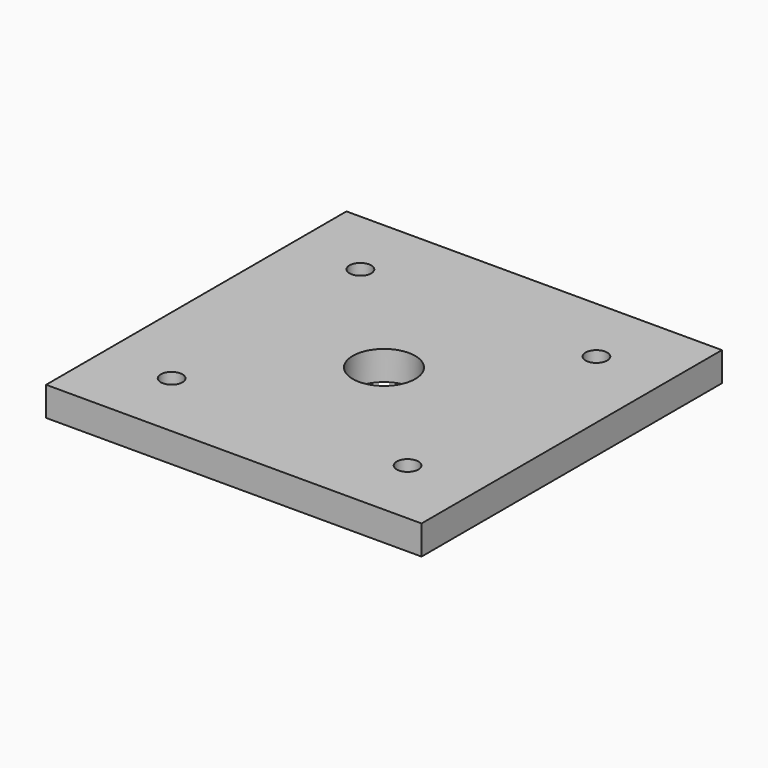
from build123d import *

# Parameters (mm, degrees)
F0_W     = 90
F0_H     = 90
F0_R     = 2.6
F0_R_2   = 2.5
F0_R_3   = 7.5
F1_DEPTH = 7
F2_DEPTH = 10


# Not quite as in the source:
# - a feature names something its author has since deleted; it is built from what else it names


with BuildPart() as f1:
    # F0 (on Top) → F1 (new body)
    with BuildSketch(Plane.XY):
        Rectangle(F0_W, F0_H)
        with Locations((-28.2842712475, -28.2842712475)):
            Circle(F0_R, mode=Mode.SUBTRACT)
        with Locations((-29.9999999986, -0.0002877)):
            Circle(F0_R_2, mode=Mode.SUBTRACT)
        with Locations((28.2842712475, -28.2842712475)):
            Circle(F0_R, mode=Mode.SUBTRACT)
        with Locations((-28.2842712475, 28.2842712475)):
            Circle(F0_R, mode=Mode.SUBTRACT)
        Circle(F0_R_3, mode=Mode.SUBTRACT)
        with Locations((29.9999999986, 0.0002877)):
            Circle(F0_R_2, mode=Mode.SUBTRACT)
        with Locations((28.2842712475, 28.2842712475)):
            Circle(F0_R, mode=Mode.SUBTRACT)
        with Locations((-29.9999999986, -0.0002877)):
            Circle(F0_R_2)
        with Locations((29.9999999986, 0.0002877)):
            Circle(F0_R_2)
    extrude(amount=F1_DEPTH)

    # F0 (on Top) → F2 (join)
    with BuildSketch(Plane.XY):
        with Locations((29.9999999986, 0.0002877)):
            Circle(F0_R_2)
        with Locations((-29.9999999986, -0.0002877)):
            Circle(F0_R_2)
    extrude(amount=-F2_DEPTH)


solid = f1.part
